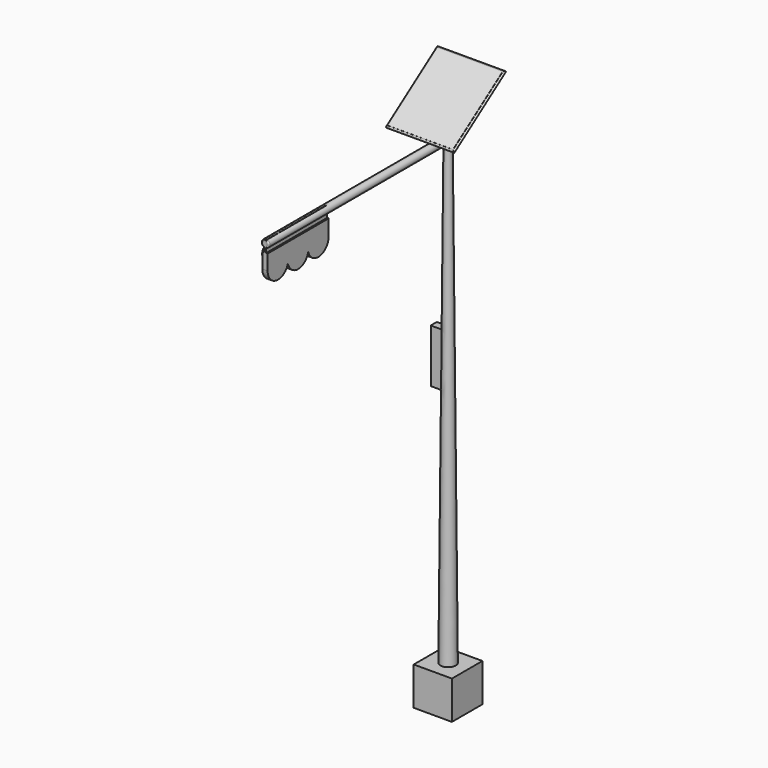
from build123d import *

# Parameters (mm, degrees)
F0_W                      = 5
F0_H                      = 5
F1_DEPTH                  = 5
F2_R                      = 1
F3_DEPTH                  = 65
F3_TAPER                  = 0.5
F8_R                      = 0.5
F9_DEPTH                  = 30
F10_W                     = 8.9562153444
F10_H                     = 10.3475067887
F11_DEPTH                 = 0.2
F12_R                     = 0.19999
F14_DEPTH                 = 0.15
F15_W                     = 10
F15_H                     = 4
F16_DEPTH                 = 0.35
F17_DEPTH                 = 1.16
DRAFT_F17_DRAFTED_ANGLE   = 11
DRAFT_F17_2_DRAFTED_ANGLE = 11
DRAFT_F17_3_DRAFTED_ANGLE = 11
F18_R                     = 1.7865180362
F19_T3_ANGLE              = 259.7960316029
F19_T7_ANGLE              = 259.7960316029
F19_T11_ANGLE             = 129.853128045
F19_T15_ANGLE             = 129.853128045
F19_T19_ANGLE             = 129.853128045
F19_T23_ANGLE             = 129.853128045
F21_DEPTH                 = 150
F22_R                     = 1.5
F23_DEPTH                 = 0.11
F26_W                     = 1
F26_H                     = 7
F27_DEPTH                 = 1
F28_W                     = 8.5562153444
F28_H                     = 9.9475067887
F29_DEPTH                 = 0.02


# Not quite as in the source:
# - a fillet or chamfer that OpenCascade refuses, or shapes differently, is made with other operations: its cross-section is extruded or revolved along the edge and cut away or added
# - a fillet or chamfer is up to 0.001 mm smaller than in the source, because OpenCascade refuses the exact size
# - an extrude with a draft is written as a straight extrude whose walls are then drafted


with BuildPart() as f1:
    # F0 (on Top) → F1 (new body)
    with BuildSketch(Plane.XY):
        Rectangle(F0_W, F0_H)
    extrude(amount=F1_DEPTH)

    # F2 (on face) → F3 (join)
    with BuildSketch(Plane.XY.offset(5)):
        Circle(F2_R)
    extrude(amount=F3_DEPTH, taper=F3_TAPER)

    # F8 (on offset) → F9 (join)
    with BuildSketch(Plane.XZ):
        with Locations((0, 65.5)):
            Circle(F8_R)
    extrude(amount=F9_DEPTH)

    # F13 (on offset) → F14 (join, symmetric)
    with BuildSketch(Plane.YZ):
        Polygon((-30, 65), (-30, 64.5), (-20, 64.5), (-20, 66), (-30, 66), align=None)
    extrude(amount=F14_DEPTH, both=True)

    # F19: fillet of radius 0.2 on 3 edges, made by hand


with BuildPart() as f11:
    # F10 (on face) → F11 (new body)
    with BuildSketch(Plane(origin=(0, -33.0459914726, 47.1945668525), x_dir=(1, 0, 0), z_dir=(0, -0.5735764364, 0.8191520443))):
        with Locations((0, 39.9303744896)):
            Rectangle(F10_W, F10_H)
    extrude(amount=F11_DEPTH)

    # F12 (radius 0.2 in the source; OpenCascade refuses exactly that, so slightly less here)
    f12_edges = [f11.edges().sort_by_distance(p)[0] for p in [
        (-4.478108, -0.451659, 70.261519),
        (0, -4.68975, 67.293976),
        (4.478108, -0.451659, 70.261519),
        (0, 3.786432, 73.229062),
    ]]
    fillet(f12_edges, radius=F12_R)


with BuildPart() as f16:
    # F15 (on offset) → F16 (new body, symmetric)
    with BuildSketch(Plane.YZ):
        with Locations((-25, 62.5)):
            Rectangle(F15_W, F15_H)
        with BuildLine():
            ThreePointArc((-29.7, 62.5), (-28.2, 64.4931122539), (-26.7, 62.5))
            ThreePointArc((-26.7, 62.5), (-28.2, 61), (-29.7, 62.5))
        make_face(mode=Mode.SUBTRACT)
        with BuildLine():
            ThreePointArc((-26.5, 62.5), (-25, 64.4931122539), (-23.5, 62.5))
            ThreePointArc((-23.5, 62.5), (-25, 61), (-26.5, 62.5))
        make_face(mode=Mode.SUBTRACT)
        with BuildLine():
            ThreePointArc((-23.3, 62.5), (-21.8, 64.4928783906), (-20.3, 62.5))
            ThreePointArc((-20.3, 62.5), (-21.8, 61), (-23.3, 62.5))
        make_face(mode=Mode.SUBTRACT)
        with BuildLine():
            ThreePointArc((-29.7, 62.5), (-28.2, 61), (-26.7, 62.5))
            ThreePointArc((-26.7, 62.5), (-28.2, 64), (-29.7, 62.5))
        make_face()
        with BuildLine():
            ThreePointArc((-29.7, 62.5), (-28.2, 64), (-26.7, 62.5))
            ThreePointArc((-26.7, 62.5), (-28.2, 64.4931122539), (-29.7, 62.5))
        make_face()
        with BuildLine():
            ThreePointArc((-26.5, 62.5), (-25, 64), (-23.5, 62.5))
            ThreePointArc((-23.5, 62.5), (-25, 64.4931122539), (-26.5, 62.5))
        make_face()
        with BuildLine():
            ThreePointArc((-23.3, 62.5), (-21.8, 64), (-20.3, 62.5))
            ThreePointArc((-20.3, 62.5), (-21.8, 64.4928783906), (-23.3, 62.5))
        make_face()
        with BuildLine():
            ThreePointArc((-26.5, 62.5), (-25, 61), (-23.5, 62.5))
            ThreePointArc((-23.5, 62.5), (-25, 64), (-26.5, 62.5))
        make_face()
        with BuildLine():
            ThreePointArc((-23.3, 62.5), (-21.8, 61), (-20.3, 62.5))
            ThreePointArc((-20.3, 62.5), (-21.8, 64), (-23.3, 62.5))
        make_face()
    extrude(amount=F16_DEPTH, both=True)


with BuildPart() as f17_drafted:
    # F15 (on offset) → F17 (new body)
    with BuildSketch(Plane.YZ):
        with BuildLine():
            ThreePointArc((-26.5, 62.5), (-25, 64), (-23.5, 62.5))
            ThreePointArc((-23.5, 62.5), (-25, 64.4931122539), (-26.5, 62.5))
        make_face()
    extrude(amount=-F17_DEPTH)

    # draft_F17_drafted
    draft_f17_drafted_walls = [f17_drafted.faces().sort_by_distance(p)[0] for p in [
        (-0.7733333333, -25, 64),
        (-0.7733333333, -25, 64.4931122539),
    ]]
    draft(draft_f17_drafted_walls, neutral_plane=Plane(origin=(0, 0, 0), x_dir=(0, 1, 0), z_dir=(-1, 0, 0)), angle=DRAFT_F17_DRAFTED_ANGLE)


with BuildPart() as f16_1:
    add(f16.part)

    # join_F17_drafted: union F17_drafted
    add(f17_drafted.part)


with BuildPart() as f17_2_drafted:
    # F15 (on offset) → F17, piece 2 (new body)
    with BuildSketch(Plane.YZ):
        with BuildLine():
            ThreePointArc((-23.3, 62.5), (-21.8, 64), (-20.3, 62.5))
            ThreePointArc((-20.3, 62.5), (-21.8, 64.4928783906), (-23.3, 62.5))
        make_face()
    extrude(amount=-F17_DEPTH)

    # draft_F17_2_drafted
    draft_f17_2_drafted_walls = [f17_2_drafted.faces().sort_by_distance(p)[0] for p in [
        (-0.7733333333, -21.8, 64),
        (-0.7733333333, -21.8, 64.4928783906),
    ]]
    draft(draft_f17_2_drafted_walls, neutral_plane=Plane(origin=(0, 0, 0), x_dir=(0, 1, 0), z_dir=(-1, 0, 0)), angle=DRAFT_F17_2_DRAFTED_ANGLE)


with BuildPart() as f16_2:
    add(f16_1.part)

    # join_F17_2_drafted: union F17_2_drafted
    add(f17_2_drafted.part)


with BuildPart() as f17_3_drafted:
    # F15 (on offset) → F17, piece 3 (new body)
    with BuildSketch(Plane.YZ):
        with BuildLine():
            ThreePointArc((-29.7, 62.5), (-28.2, 64), (-26.7, 62.5))
            ThreePointArc((-26.7, 62.5), (-28.2, 64.4931122539), (-29.7, 62.5))
        make_face()
    extrude(amount=-F17_DEPTH)

    # draft_F17_3_drafted
    draft_f17_3_drafted_walls = [f17_3_drafted.faces().sort_by_distance(p)[0] for p in [
        (-0.7733333333, -28.2, 64),
        (-0.7733333333, -28.2, 64.4931122539),
    ]]
    draft(draft_f17_3_drafted_walls, neutral_plane=Plane(origin=(0, 0, 0), x_dir=(0, 1, 0), z_dir=(-1, 0, 0)), angle=DRAFT_F17_3_DRAFTED_ANGLE)


with BuildPart() as f16_3:
    add(f16_2.part)

    # join_F17_3_drafted: union F17_3_drafted
    add(f17_3_drafted.part)

    # F18
    f18_edges = [f16_3.edges().sort_by_distance(p)[0] for p in [
        (0, -20, 60.5),
        (0, -30, 60.5),
    ]]
    fillet(f18_edges, radius=F18_R)

    # F20 (on face) → F21 (cut, symmetric)
    with BuildSketch(Plane(origin=(-0.35, 0, 0), x_dir=(0, -1, 0), z_dir=(-1, 0, 0))):
        with BuildLine():
            Line((20, 62.382313551), (20, 62.4798834324))
            ThreePointArc((20, 62.4798834324), (19.9992998645, 62.4310984917), (20, 62.382313551))
        make_face()
        with BuildLine():
            ThreePointArc((23.348921888, 62.0203100063), (21.5166017158, 60.7409442424), (20, 62.382313551))
            Line((20, 62.382313551), (20, 62.2865180362))
            ThreePointArc((20, 62.2865180362), (20.5232590181, 61.0232590181), (21.7865180362, 60.5))
            Line((21.7865180362, 60.5), (28.2134819638, 60.5))
            ThreePointArc((28.2134819638, 60.5), (29.4767409819, 61.0232590181), (30, 62.2865180362))
            Line((30, 62.2865180362), (30, 62.5042021275))
            ThreePointArc((30, 62.5042021275), (28.5444608935, 60.8205911402), (26.6699437052, 62.0203100063))
            ThreePointArc((26.6699437052, 62.0203100063), (25.0094327966, 60.6845949531), (23.348921888, 62.0203100063))
        make_face()
    extrude(amount=F21_DEPTH, both=True, mode=Mode.SUBTRACT)


with BuildPart() as f19_tool1:
    # F19_s2 → F19_t3 (revolve)
    with BuildSketch(Plane(origin=(-32.2320043993, 0, 26.9482423006), x_dir=(0, 1, 0), z_dir=(0.7671873653, 0, -0.6414230636))):
        with BuildLine():
            ThreePointArc((-29.8, 50.750772425), (-29.9414213562, 50.6921937813), (-30, 50.550772425))
            Line((-30, 50.550772425), (-30, 50.750772425))
            Line((-30, 50.750772425), (-29.8, 50.750772425))
        make_face()
    revolve(axis=Axis((0, -30, 65.5), (0, -1, 0)), revolution_arc=F19_T3_ANGLE)

    split(bisect_by=Plane.YZ.offset(0.15), keep=Keep.TOP)


with BuildPart() as f19_tool5:
    # F19_s6 → F19_t7 (revolve)
    with BuildSketch(Plane(origin=(-32.2320043993, 0, 26.9482423006), x_dir=(0, 1, 0), z_dir=(0.7671873653, 0, -0.6414230636))):
        with BuildLine():
            ThreePointArc((-29.8, 50.750772425), (-29.9414213562, 50.6921937813), (-30, 50.550772425))
            Line((-30, 50.550772425), (-30, 50.750772425))
            Line((-30, 50.750772425), (-29.8, 50.750772425))
        make_face()
    revolve(axis=Axis((0, -30, 65.5), (0, -1, 0)), revolution_arc=F19_T7_ANGLE)

    split(bisect_by=Plane.YZ.offset(-0.15), keep=Keep.BOTTOM)


with BuildPart() as f19_tool9:
    # F19_s10 → F19_t11 (revolve)
    with BuildSketch(Plane(origin=(-32.2228741883, 0, 26.8977458153), x_dir=(0, 1, 0), z_dir=(-0.7676896457, 0, 0.6408218222))):
        with BuildLine():
            ThreePointArc((-29.8, -49.7836717941), (-29.9414213562, -49.8422504378), (-30, -49.9836717941))
            Line((-30, -49.9836717941), (-30, -49.7836717941))
            Line((-30, -49.7836717941), (-29.8, -49.7836717941))
        make_face()
    revolve(axis=Axis((0, -30, 65.5), (0, -1, 0)), revolution_arc=F19_T11_ANGLE)

    split(bisect_by=Plane.YZ.offset(-0.15), keep=Keep.BOTTOM)


with BuildPart() as f19_tool13:
    # F19_s14 → F19_t15 (revolve)
    with BuildSketch(Plane(origin=(-32.2228741883, 0, 26.8977458153), x_dir=(0, 1, 0), z_dir=(-0.7676896457, 0, 0.6408218222))):
        with BuildLine():
            ThreePointArc((-29.8, -49.7836717941), (-29.9414213562, -49.8422504378), (-30, -49.9836717941))
            Line((-30, -49.9836717941), (-30, -49.7836717941))
            Line((-30, -49.7836717941), (-29.8, -49.7836717941))
        make_face()
    revolve(axis=Axis((0, -30, 65.5), (0, -1, 0)), revolution_arc=F19_T15_ANGLE)

    split(bisect_by=Plane.YZ.offset(0.15), keep=Keep.TOP)


with BuildPart() as f19_tool17:
    # F19_s18 → F19_t19 (revolve)
    with BuildSketch(Plane.XY.offset(65.5)):
        with BuildLine():
            ThreePointArc((0.5, -29.8), (0.4414213562, -29.9414213562), (0.3, -30))
            Line((0.3, -30), (0.5, -30))
            Line((0.5, -30), (0.5, -29.8))
        make_face()
    revolve(axis=Axis((0, -30, 65.5), (0, -1, 0)), revolution_arc=F19_T19_ANGLE)

    split(bisect_by=Plane.YZ.offset(0.15), keep=Keep.TOP)


with BuildPart() as f19_tool21:
    # F19_s22 → F19_t23 (revolve)
    with BuildSketch(Plane.XY.offset(65.5)):
        with BuildLine():
            ThreePointArc((0.5, -29.8), (0.4414213562, -29.9414213562), (0.3, -30))
            Line((0.3, -30), (0.5, -30))
            Line((0.5, -30), (0.5, -29.8))
        make_face()
    revolve(axis=Axis((0, -30, 65.5), (0, -1, 0)), revolution_arc=F19_T23_ANGLE)

    split(bisect_by=Plane.YZ.offset(-0.15), keep=Keep.BOTTOM)


with BuildPart() as f1_1:
    add(f1.part)

    # F19_t25: cut F19_tool1, F19_tool5, F19_tool9, F19_tool13, F19_tool17, F19_tool21
    add([f19_tool1.part, f19_tool5.part, f19_tool9.part, f19_tool13.part, f19_tool17.part, f19_tool21.part], mode=Mode.SUBTRACT)

    # F26 (on offset) → F27 (join, symmetric)
    with BuildSketch(Plane(origin=(-0.87, 0, 0), x_dir=(0, -1, 0), z_dir=(-1, 0, 0))):
        with Locations((0, 40)):
            Rectangle(F26_W, F26_H)
    extrude(amount=F27_DEPTH, both=True)


with BuildPart() as f23:
    # F22 (on face) → F23 (new body, symmetric)
    with BuildSketch(Plane(origin=(-0.35, 0, 0), x_dir=(0, -1, 0), z_dir=(-1, 0, 0))):
        with Locations((21.8, 62.5)):
            Circle(F22_R)
    extrude(amount=F23_DEPTH, both=True)


with BuildPart() as f23b:
    # F22 (on face) → F23, piece 2 (new body, symmetric)
    with BuildSketch(Plane(origin=(-0.35, 0, 0), x_dir=(0, -1, 0), z_dir=(-1, 0, 0))):
        with Locations((25, 62.5)):
            Circle(F22_R)
    extrude(amount=F23_DEPTH, both=True)


with BuildPart() as f23c:
    # F22 (on face) → F23, piece 3 (new body, symmetric)
    with BuildSketch(Plane(origin=(-0.35, 0, 0), x_dir=(0, -1, 0), z_dir=(-1, 0, 0))):
        with Locations((28.2, 62.5)):
            Circle(F22_R)
    extrude(amount=F23_DEPTH, both=True)


with BuildPart() as f29:
    # F28 (on face) → F29 (new body)
    with BuildSketch(Plane(origin=(0, -33.1607067599, 47.3583972613), x_dir=(1, 0, 0), z_dir=(0, -0.5735764364, 0.8191520443))):
        with Locations((0, 39.9303744896)):
            Rectangle(F28_W, F28_H)
    extrude(amount=F29_DEPTH)


solid = Compound([f11.part, f16_3.part, f1_1.part, f23.part, f23b.part, f23c.part, f29.part])
